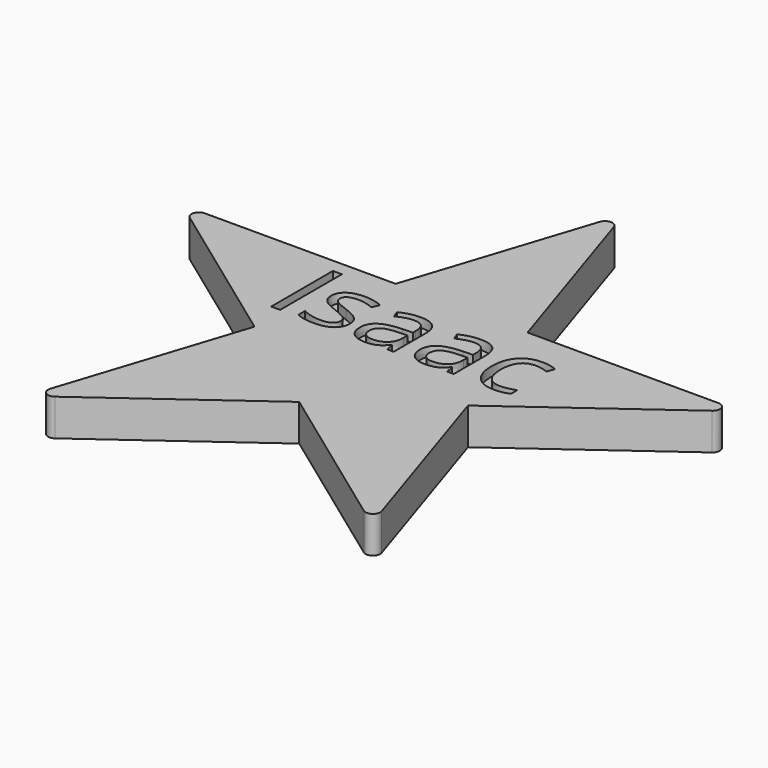
from build123d import *

# Parameters (mm, degrees)
F1_DEPTH     = 6.35
F2_R         = 1.27
F3_TEXT_SIZE = 18.6940275591
F4_DEPTH     = 1.5875


# Not quite as in the source:
# - Text() gives the source's letters only with a copy of the font that has no kerning and outlines rounded to 1/6400 em; it was checked with that copy


with BuildPart() as f1:
    # F0 (on Top) → F1 (new body)
    with BuildSketch(Plane.XY):
        Polygon((-18.4541802113, -5.9961266285), (-29.8594908165, -41.0980633142), (0, -19.4038733715), align=None)
        Polygon((-11.4053106051, 15.6980633142), (-48.3136710278, 15.6980633142), (-18.4541802113, -5.9961266285), align=None)
        Polygon((11.4053106051, 15.6980633142), (0, 50.8), (-11.4053106051, 15.6980633142), align=None)
        Polygon((11.4053106051, 15.6980633142), (-11.4053106051, 15.6980633142), (-18.4541802113, -5.9961266285), (0, -19.4038733715), (18.4541802113, -5.9961266285), align=None)
        Polygon((18.4541802113, -5.9961266285), (48.3136710278, 15.6980633142), (11.4053106051, 15.6980633142), align=None)
        Polygon((0, -19.4038733715), (29.8594908165, -41.0980633142), (18.4541802113, -5.9961266285), align=None)
    extrude(amount=F1_DEPTH)

    # F2
    f2_edges = [f1.edges().sort_by_distance(p)[0] for p in [
        (-29.859491, -41.098063, 3.175),
        (29.859491, -41.098063, 3.175),
        (48.313671, 15.698063, 3.175),
        (0, 50.8, 3.175),
        (-48.313671, 15.698063, 3.175),
    ]]
    fillet(f2_edges, radius=F2_R)

    # F3 (on face) → F4 (cut)
    with BuildSketch(Plane.XY.offset(6.35)):
        with Locations((-22.2049996101, 0)):
            Text('Isaac', F3_TEXT_SIZE, font='Open Sans', text_align=(TextAlign.LEFT, TextAlign.BOTTOM))
    extrude(amount=-F4_DEPTH, mode=Mode.SUBTRACT)


solid = f1.part
